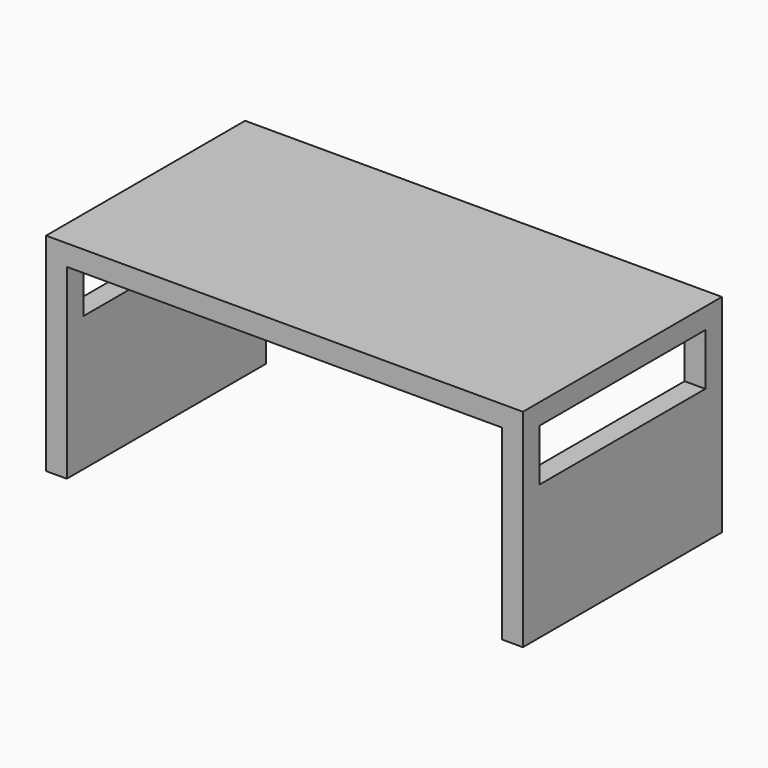
from build123d import *

# Parameters (mm, degrees)
F0_W     = 575
F0_H     = 300
F1_DEPTH = 50
F2_W     = 50
F2_H     = 300
F3_DEPTH = 450
F5_DEPTH = 50
F8_W     = 500
F8_H     = 125
F9_DEPTH = 1150.001


# Not quite as in the source:
# - a feature of the source that left no trace in its solid (it failed there, or was rolled back) is left out


with BuildPart() as f1:
    # F0 (on Top) → F1 (new body)
    with BuildSketch(Plane.XY):
        with Locations((287.5, -150)):
            Rectangle(F0_W, F0_H)
    extrude(amount=-F1_DEPTH)

    # F2 (on face) → F3 (join)
    with BuildSketch(Plane(origin=(0, 0, -50), x_dir=(1, 0, 0), z_dir=(0, 0, -1))):
        with Locations((550, 150)):
            Rectangle(F2_W, F2_H)
    extrude(amount=F3_DEPTH)

    # F4 (on face) → F5 (join, through all)
    with BuildSketch(Plane.YZ.offset(575)):
        Polygon((50, -30), (0, -80), (0, -150.7106781187), (120.7106781187, -30), align=None)
    extrude(amount=-F5_DEPTH)

    # F6: F1 across plane


with BuildPart() as f1_1:
    add(f1.part)
    add(f1.part.mirror(Plane.YZ))

    # F7: F1 across plane


with BuildPart() as f1_2:
    add(f1_1.part)
    add(f1_1.part.mirror(Plane.XZ))

    # F8 (on face) → F9 (cut, through all)
    with BuildSketch(Plane.YZ.offset(575)):
        with Locations((0, -112.5)):
            Rectangle(F8_W, F8_H)
    extrude(amount=-F9_DEPTH, mode=Mode.SUBTRACT)


solid = f1_2.part
